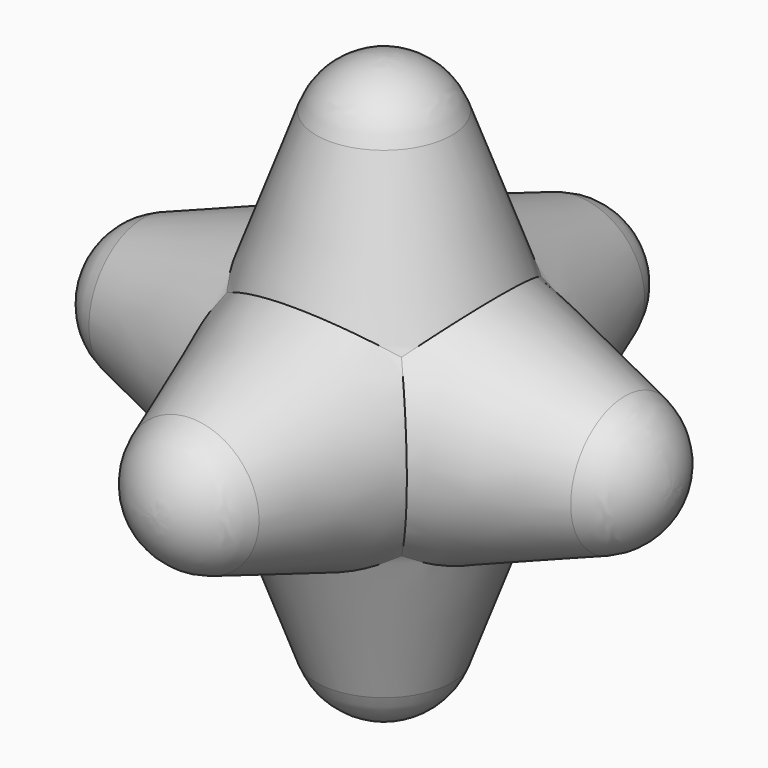
from build123d import *

# Parameters (mm, degrees)
F3_ANGLE = 90
F4_ANGLE = -90
F5_COUNT = 4


with BuildPart() as f1:
    # F0 (on Front) → F1 (revolve)
    with BuildSketch(Plane.XZ):
        with BuildLine():
            Line((0, 0), (0, 20))
            ThreePointArc((0, 20), (-2.867882, 19.09576), (-4.698463, 16.710101))
            Line((-4.698463, 16.710101), (-10.780442, 0))
            Line((-10.780442, 0), (0, 0))
        make_face()
    revolve(axis=Axis((0, 0, 10), (0, 0, -1)))


with BuildPart() as f3_1:
    # F3: copy of F1
    add(f1.part.rotate(Axis((0, -13.434995, 0), (0, -1, 0)), F3_ANGLE))


with BuildPart() as f4_1:
    # F4: copy of F1
    add(f1.part.rotate(Axis((0, -13.434995, 0), (0, -1, 0)), F4_ANGLE))


with BuildPart() as f1_1:
    add(f1.part)

    add(f3_1.part)  # F5 merges F3_1

    add(f4_1.part)  # F5 merges F4_1
    # F5: F1 ×4 about axis
    f5_axis = Axis((22.578118, 0, 0), (1, 0, 0))
    for i in range(1, F5_COUNT):
        add(f1.part.rotate(f5_axis, i * 360 / F5_COUNT))


solid = f1_1.part
